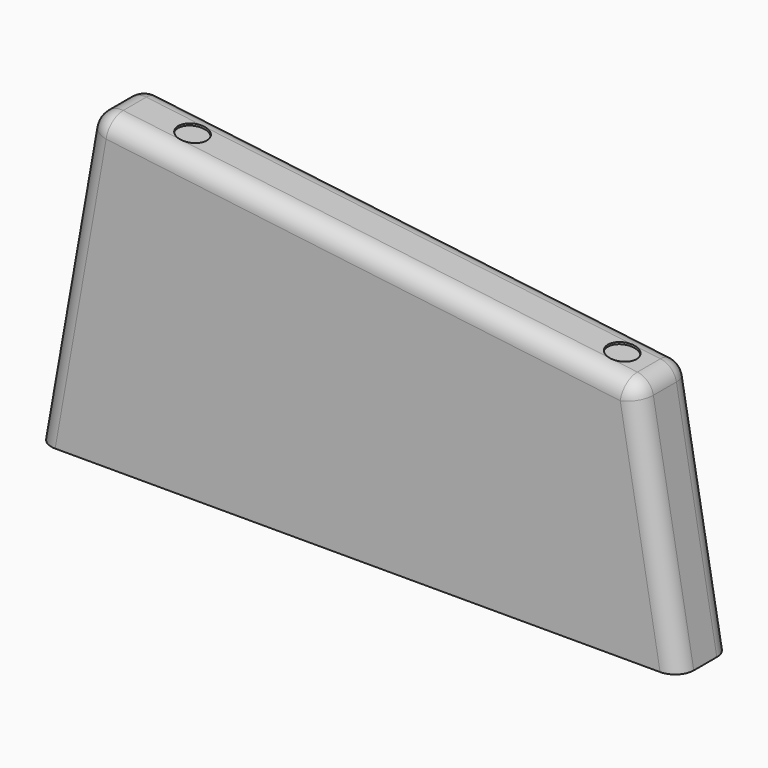
from build123d import *

# Parameters (mm, degrees)
F1_DEPTH = 16
F2_R     = 3.5
F3_DEPTH = 0.5
F4_R     = 4.49999


# Not quite as in the source:
# - a fillet or chamfer is up to 0.001 mm smaller than in the source, because OpenCascade refuses the exact size


with BuildPart() as f1:
    # F0 (on Front) → F1 (new body)
    with BuildSketch(Plane.XZ):
        Polygon((-56.24990897, 75.1608516625), (-69.5027950111, 0), (86.4972049889, 0), (76.1099402454, 58.9091056954), align=None)
    extrude(amount=F1_DEPTH)

    # F2 (on face) → F3 (cut)
    with BuildSketch(Plane(origin=(8.256096508, 0, 67.2405101043), x_dir=(0.9925461516, 0, -0.1218693434), z_dir=(0.1218693434, 0, 0.9925461516))):
        with Locations((-46.5904343202, -8)):
            Circle(F2_R)
        with Locations((58.5095656798, -8)):
            Circle(F2_R)
    extrude(amount=-F3_DEPTH, mode=Mode.SUBTRACT)

    # F4 (radius 4.5 in the source; OpenCascade refuses exactly that, so slightly less here)
    f4_edges = [f1.edges().sort_by_distance(p)[0] for p in [
        (9.930016, -16, 67.034979),
        (9.930016, 0, 67.034979),
        (81.303573, 0, 29.454553),
        (81.303573, -16, 29.454553),
        (-62.876352, -16, 37.580426),
        (-62.876352, 0, 37.580426),
        (-56.249909, -8, 75.160852),
        (76.10994, -8, 58.909106),
    ]]
    fillet(f4_edges, radius=F4_R)


solid = f1.part
